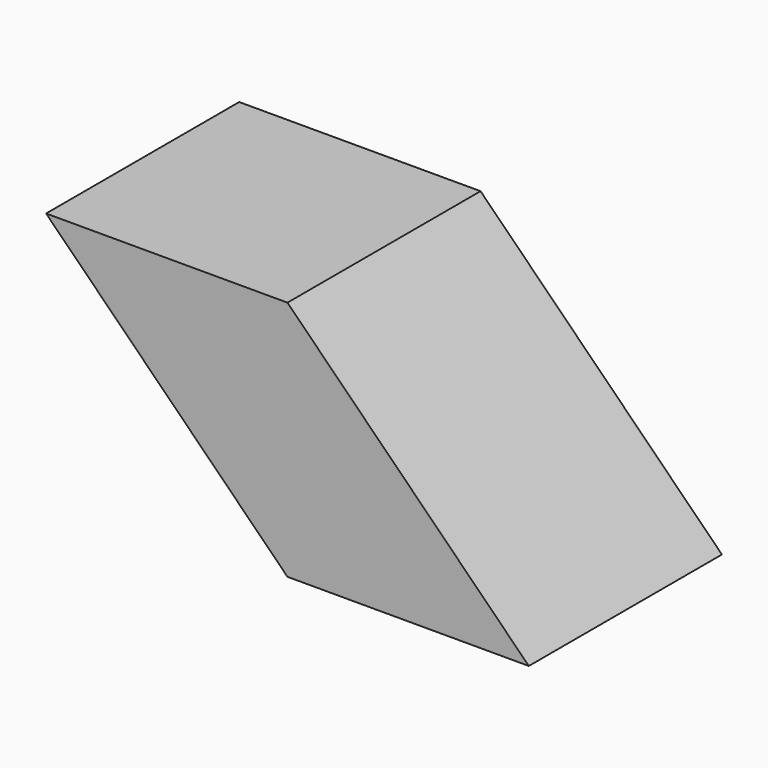
from build123d import *

# Parameters (mm, degrees)
F1_DEPTH = 16
F2_SIZE  = 15.99999


# Not quite as in the source:
# - a fillet or chamfer is up to 0.001 mm smaller than in the source, because OpenCascade refuses the exact size


with BuildPart() as f1:
    # F0 (on Top) → F1 (new body)
    with BuildSketch(Plane.XY):
        Polygon((8, -8), (8, 8), (0, 8), (-8, 8), (-16, 8), (-24, 8), (-24, -8), (-16, -8), (-8, -8), (0, -8), align=None)
    extrude(amount=F1_DEPTH)

    # F2 (size 16 in the source; OpenCascade refuses exactly that, so slightly less here)
    f2_edges = [f1.edges().sort_by_distance(p)[0] for p in [
        (8, 0, 16),
        (-24, 0, 0),
    ]]
    chamfer(f2_edges, length=F2_SIZE)


solid = f1.part
